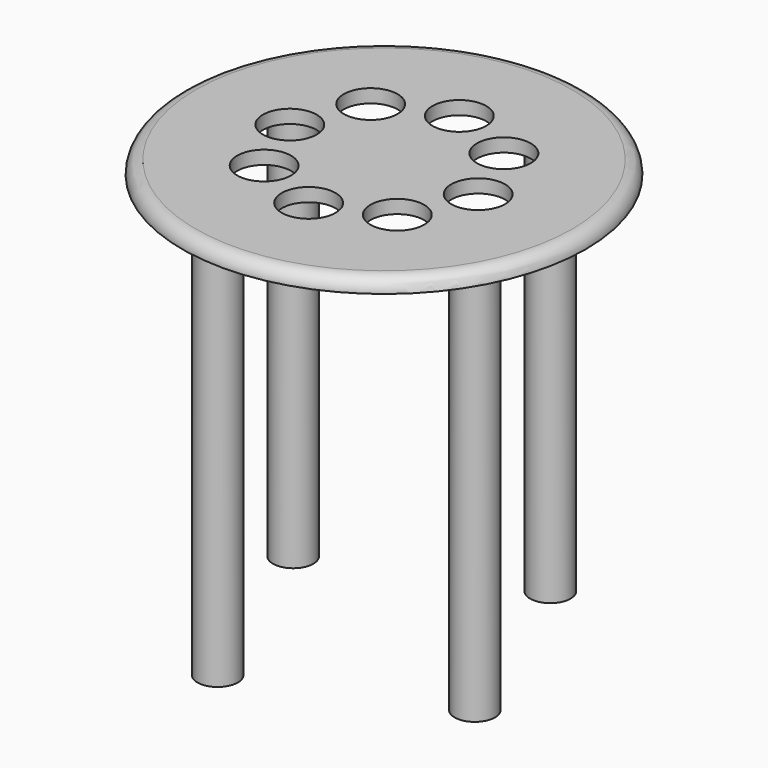
from build123d import *

# Parameters (mm, degrees)
F0_R     = 75
F0_R_2   = 10
F1_DEPTH = 5
F2_R     = 4.99999
F3_R     = 7.5
F4_DEPTH = 150


# Not quite as in the source:
# - a fillet or chamfer is up to 0.001 mm smaller than in the source, because OpenCascade refuses the exact size


with BuildPart() as f1:
    # F0 (on Top) → F1 (new body)
    with BuildSketch(Plane.XY):
        Circle(F0_R)
        with Locations((-24.7487373415, -24.7487373415)):
            Circle(F0_R_2, mode=Mode.SUBTRACT)
        with Locations((0, -35)):
            Circle(F0_R_2, mode=Mode.SUBTRACT)
        with Locations((24.7487373415, -24.7487373415)):
            Circle(F0_R_2, mode=Mode.SUBTRACT)
        with Locations((-35, 0)):
            Circle(F0_R_2, mode=Mode.SUBTRACT)
        with Locations((-24.7487373415, 24.7487373415)):
            Circle(F0_R_2, mode=Mode.SUBTRACT)
        with Locations((35, 0)):
            Circle(F0_R_2, mode=Mode.SUBTRACT)
        with Locations((0, 35)):
            Circle(F0_R_2, mode=Mode.SUBTRACT)
        with Locations((24.7487373415, 24.7487373415)):
            Circle(F0_R_2, mode=Mode.SUBTRACT)
    extrude(amount=F1_DEPTH)

    # F2 (radius 5 in the source; OpenCascade refuses exactly that, so slightly less here)
    f2_edges = [f1.edges().sort_by_distance(p)[0] for p in [
        (-75, 0, 5),
    ]]
    fillet(f2_edges, radius=F2_R)

    # F3 (on face) → F4 (join)
    with BuildSketch(Plane.XY):
        with Locations((21.2406198754, 50.7329879596)):
            Circle(F3_R)
        with Locations((-50.7329879596, 21.2406198754)):
            Circle(F3_R)
        with Locations((-21.2406198754, -50.7329879596)):
            Circle(F3_R)
        with Locations((50.7329879596, -21.2406198754)):
            Circle(F3_R)
    extrude(amount=-F4_DEPTH)


solid = f1.part
